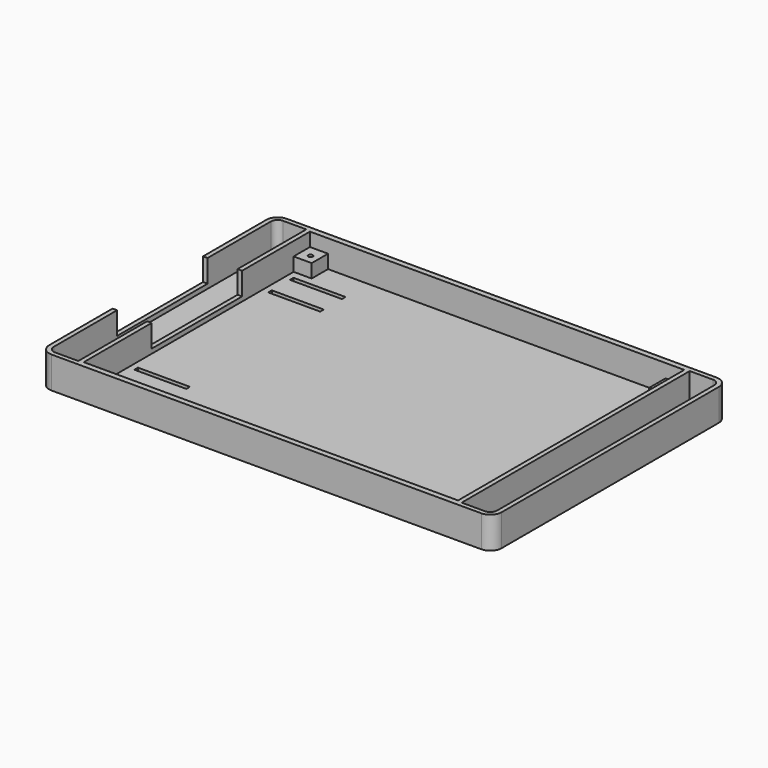
from build123d import *

# Parameters (mm, degrees)
F0_W         = 200
F0_H         = 130
F0_W_2       = 0.3
F0_H_2       = 106.96
F1_DEPTH     = 2
F2_DEPTH     = 14
F3_DEPTH     = 8
F4_D         = 2
F5_R         = 5
F6_T         = 2
F6_T3_DEPTH  = 16
F6_T5_DEPTH  = 10
F6_T7_DEPTH  = 12
F6_T9_DEPTH  = 10
F6_T11_DEPTH = 153.2
F6_T13_DEPTH = 12
F6_T15_DEPTH = 4.3
F6_T17_DEPTH = 129
F6_T19_DEPTH = 12.3
F6_T21_DEPTH = 11.7
F6_T23_DEPTH = 153.2
F6_T25_DEPTH = 13.02
F6_T27_DEPTH = 13.02
F6_T29_DEPTH = 110.96
F7_W         = 23
F7_H         = 2
F8_DEPTH     = 22.5
F9_W         = 50
F9_H         = 8
F9_H_2       = 2
F10_DEPTH    = 25


# Not quite as in the source:
# - a shell that OpenCascade refuses in one call is made with other operations: the cavity is built on its own and cut out


with BuildPart() as f1:
    # F0 (on Top) → F1 (new body)
    with BuildSketch(Plane.XY):
        Rectangle(F0_W, F0_H)
        Polygon((77.15, 62.5), (79.15, 62.5), (82.45, 62.5), (82.75, 62.5), (82.75, 59.5), (82.75, -58.77), (82.75, -62.5), (82.45, -62.5), (79.45, -62.5), (77.45, -62.5), (74.75, -62.5), (-74.45, -62.5), (-77.45, -62.5), (-79.45, -62.5), (-82.75, -62.5), (-82.75, -58.77), (-82.75, -53.48), (-82.75, 53.48), (-82.75, 59.5), (-82.75, 62.5), (-79.75, 62.5), (-77.75, 62.5), (-74.75, 62.5), (74.45, 62.5), align=None, mode=Mode.SUBTRACT)
        Polygon((74.45, 53.48), (74.45, 62.5), (-74.75, 62.5), (-74.75, 53.48), (-82.45, 53.48), (-82.45, -53.48), (-74.45, -53.48), (-74.45, -62.5), (74.75, -62.5), (74.75, -53.48), (82.45, -53.48), (82.45, 53.48), align=None)
        Polygon((-74.75, 53.48), (-74.75, 62.5), (-77.75, 62.5), (-79.75, 62.5), (-82.75, 62.5), (-82.75, 59.5), (-82.75, 53.48), (-82.45, 53.48), align=None)
        Polygon((82.45, 62.5), (79.15, 62.5), (77.15, 62.5), (74.45, 62.5), (74.45, 53.48), (82.45, 53.48), align=None)
        Polygon((82.45, -62.5), (82.45, -53.48), (74.75, -53.48), (74.75, -62.5), (77.45, -62.5), (79.45, -62.5), align=None)
        Polygon((-74.45, -53.48), (-82.45, -53.48), (-82.75, -53.48), (-82.75, -58.77), (-82.75, -62.5), (-79.45, -62.5), (-77.45, -62.5), (-74.45, -62.5), align=None)
        with Locations((-82.6, 0)):
            Rectangle(F0_W_2, F0_H_2)
        Polygon((82.75, 62.5), (82.45, 62.5), (82.45, 53.48), (82.45, -53.48), (82.45, -62.5), (82.75, -62.5), (82.75, -58.77), (82.75, 59.5), align=None)
    extrude(amount=F1_DEPTH)

    # F0 (on Top) → F2 (join)
    with BuildSketch(Plane.XY):
        Rectangle(F0_W, F0_H)
        Polygon((77.15, 62.5), (79.15, 62.5), (82.45, 62.5), (82.75, 62.5), (82.75, 59.5), (82.75, -58.77), (82.75, -62.5), (82.45, -62.5), (79.45, -62.5), (77.45, -62.5), (74.75, -62.5), (-74.45, -62.5), (-77.45, -62.5), (-79.45, -62.5), (-82.75, -62.5), (-82.75, -58.77), (-82.75, -53.48), (-82.75, 53.48), (-82.75, 59.5), (-82.75, 62.5), (-79.75, 62.5), (-77.75, 62.5), (-74.75, 62.5), (74.45, 62.5), align=None, mode=Mode.SUBTRACT)
    extrude(amount=F2_DEPTH)

    # F0 (on Top) → F3 (join)
    with BuildSketch(Plane.XY):
        Polygon((-74.45, -53.48), (-82.45, -53.48), (-82.75, -53.48), (-82.75, -58.77), (-82.75, -62.5), (-79.45, -62.5), (-77.45, -62.5), (-74.45, -62.5), align=None)
        Polygon((-74.75, 53.48), (-74.75, 62.5), (-77.75, 62.5), (-79.75, 62.5), (-82.75, 62.5), (-82.75, 59.5), (-82.75, 53.48), (-82.45, 53.48), align=None)
        Polygon((82.45, -62.5), (82.45, -53.48), (74.75, -53.48), (74.75, -62.5), (77.45, -62.5), (79.45, -62.5), align=None)
        Polygon((82.45, 62.5), (79.15, 62.5), (77.15, 62.5), (74.45, 62.5), (74.45, 53.48), (82.45, 53.48), align=None)
    extrude(amount=F3_DEPTH)

    # F4 (through all)
    with Locations(Plane(origin=(0, 0, 0), x_dir=(1, 0, 0), z_dir=(0, 0, -1))):
        with Locations((-78.45, 57.48), (78.45, 57.48), (-78.45, -57.48), (78.45, -57.48)):
            Hole(F4_D / 2)

    # F5
    f5_edges = [f1.edges().sort_by_distance(p)[0] for p in [
        (-100, -65, 7),
        (-100, 65, 7),
        (100, 65, 7),
        (100, -65, 7),
    ]]
    fillet(f5_edges, radius=F5_R)

    # F6: shell of thickness 2, made by hand


with BuildPart() as f6_core1:
    # F6_t2: copy of F1
    add(f1.part)

    # the walls: a layer under each face that stays
    f6_faces = [f6_core1.faces().sort_by_distance(p)[0] for p in [
        (100, 0, 7),
        (98.5355339059, -63.5355339059, 7),
        (98.5355339059, 63.5355339059, 7),
        (0, 0, 0),
        (0, -65, 7),
        (0, 65, 7),
        (-98.5355339059, -63.5355339059, 7),
        (-98.5355339059, 63.5355339059, 7),
        (-100, 0, 7),
        (0, 62.5, 8),
        (82.75, 0, 8),
        (0, -62.5, 8),
        (-82.75, 0, 8),
        (-79.45, -57.48, 4),
        (77.45, -57.48, 4),
        (-79.45, 57.48, 4),
        (77.45, 57.48, 4),
        (-81.4166666667, 54.9833333333, 8),
        (-74.75, 57.99, 5),
        (0, 0, 2),
        (74.45, 57.99, 5),
        (75.7833333333, 54.9833333333, 8),
        (82.45, 57.99, 5),
        (-74.45, -57.99, 5),
        (-81.3666666667, -60.9966666667, 8),
        (82.45, -57.99, 5),
        (76.0333333333, -60.9966666667, 8),
        (74.75, -57.99, 5),
        (-78.75, 53.48, 5),
        (-78.6, -53.48, 5),
        (78.6, -53.48, 5),
        (78.45, 53.48, 5),
    ]]
    thicken(f6_faces, amount=-F6_T, mode=Mode.SUBTRACT)

    # F6_s4 → F6_t3 (cut)
    with BuildSketch(Plane.XY):
        Polygon((82.73, 62.48), (82.75, 64.5), (84.75, 64.5), (84.75, 62.5), align=None)
        Polygon((82.73, -62.48), (84.75, -62.5), (84.75, -64.5), (82.75, -64.5), align=None)
    extrude(amount=F6_T3_DEPTH, mode=Mode.SUBTRACT)

    # F6_s6 → F6_t5 (cut)
    with BuildSketch(Plane.XY.offset(6)):
        Polygon((-82.73, 62.48), (-82.75, 64.5), (-84.75, 64.5), (-84.75, 62.5), align=None)
        Polygon((-82.73, -62.48), (-82.75, -64.5), (-84.75, -64.5), (-84.75, -62.5), align=None)
    extrude(amount=F6_T5_DEPTH, mode=Mode.SUBTRACT)

    # F6_s8 → F6_t7 (cut)
    with BuildSketch(Plane.YZ.offset(-84.75)):
        Polygon((62.48, 8.02), (64.5, 8), (64.5, 6), (62.5, 6), align=None)
        Polygon((53.46, 2.02), (53.48, 0), (55.48, 0), (55.48, 2), align=None)
    extrude(amount=F6_T7_DEPTH, mode=Mode.SUBTRACT)

    # F6_s10 → F6_t9 (cut)
    with BuildSketch(Plane.XY):
        Polygon((-74.73, 62.48), (-74.75, 64.5), (-76.75, 64.5), (-76.75, 62.5), align=None)
        Polygon((74.43, 62.48), (74.45, 64.5), (76.45, 64.5), (76.45, 62.5), align=None)
        Polygon((82.47, 62.48), (82.45, 64.5), (80.45, 64.5), (80.45, 62.5), align=None)
        Polygon((-74.43, -62.48), (-74.45, -64.5), (-76.45, -64.5), (-76.45, -62.5), align=None)
        Polygon((82.47, -62.48), (82.45, -64.5), (80.45, -64.5), (80.45, -62.5), align=None)
        Polygon((74.73, -62.48), (74.75, -64.5), (76.75, -64.5), (76.75, -62.5), align=None)
        Polygon((-82.73, 53.46), (-84.75, 53.48), (-84.75, 55.48), (-82.75, 55.48), align=None)
        Polygon((-82.73, -53.46), (-84.75, -53.48), (-84.75, -55.48), (-82.75, -55.48), align=None)
    extrude(amount=F6_T9_DEPTH, mode=Mode.SUBTRACT)

    # F6_s12 → F6_t11 (cut)
    with BuildSketch(Plane.YZ.offset(-76.75)):
        Polygon((62.48, 2.02), (64.5, 2), (64.5, 0), (62.5, 0), align=None)
    extrude(amount=F6_T11_DEPTH, mode=Mode.SUBTRACT)

    # F6_s14 → F6_t13 (cut)
    with BuildSketch(Plane.YZ.offset(72.45)):
        Polygon((62.48, 8.02), (64.5, 8), (64.5, 6), (62.5, 6), align=None)
        Polygon((53.46, 2.02), (53.48, 0), (55.48, 0), (55.48, 2), align=None)
    extrude(amount=F6_T13_DEPTH, mode=Mode.SUBTRACT)

    # F6_s16 → F6_t15 (cut)
    with BuildSketch(Plane.YZ.offset(80.45)):
        Polygon((62.48, 2.02), (64.5, 2), (64.5, 0), (62.5, 0), align=None)
        Polygon((-62.48, 2.02), (-64.5, 2), (-64.5, 0), (-62.5, 0), align=None)
    extrude(amount=F6_T15_DEPTH, mode=Mode.SUBTRACT)

    # F6_s18 → F6_t17 (cut)
    with BuildSketch(Plane.XZ.offset(-64.5)):
        Polygon((82.73, 2.02), (84.75, 2), (84.75, 0), (82.75, 0), align=None)
    extrude(amount=F6_T17_DEPTH, mode=Mode.SUBTRACT)

    # F6_s20 → F6_t19 (cut)
    with BuildSketch(Plane.YZ.offset(-84.75)):
        Polygon((-62.48, 8.02), (-64.5, 8), (-64.5, 6), (-62.5, 6), align=None)
        Polygon((-53.46, 2.02), (-53.48, 0), (-55.48, 0), (-55.48, 2), align=None)
    extrude(amount=F6_T19_DEPTH, mode=Mode.SUBTRACT)

    # F6_s22 → F6_t21 (cut)
    with BuildSketch(Plane.YZ.offset(72.75)):
        Polygon((-62.48, 8.02), (-64.5, 8), (-64.5, 6), (-62.5, 6), align=None)
        Polygon((-53.46, 2.02), (-53.48, 0), (-55.48, 0), (-55.48, 2), align=None)
    extrude(amount=F6_T21_DEPTH, mode=Mode.SUBTRACT)

    # F6_s24 → F6_t23 (cut)
    with BuildSketch(Plane.YZ.offset(-76.45)):
        Polygon((-62.48, 2.02), (-64.5, 2), (-64.5, 0), (-62.5, 0), align=None)
    extrude(amount=F6_T23_DEPTH, mode=Mode.SUBTRACT)

    # F6_s26 → F6_t25 (cut)
    with BuildSketch(Plane.XZ.offset(-64.5)):
        Polygon((-82.73, 8.02), (-84.75, 8), (-84.75, 6), (-82.75, 6), align=None)
        Polygon((-74.73, 2.02), (-76.75, 2), (-76.75, 0), (-74.75, 0), align=None)
        Polygon((74.43, 2.02), (74.45, 0), (76.45, 0), (76.45, 2), align=None)
        Polygon((82.47, 2.02), (82.45, 0), (80.45, 0), (80.45, 2), align=None)
    extrude(amount=F6_T25_DEPTH, mode=Mode.SUBTRACT)

    # F6_s28 → F6_t27 (cut)
    with BuildSketch(Plane.XZ.offset(51.48)):
        Polygon((-82.73, 8.02), (-84.75, 8), (-84.75, 6), (-82.75, 6), align=None)
        Polygon((82.47, 2.02), (82.45, 0), (80.45, 0), (80.45, 2), align=None)
        Polygon((74.73, 2.02), (74.75, 0), (76.75, 0), (76.75, 2), align=None)
        Polygon((-74.43, 2.02), (-74.45, 0), (-76.45, 0), (-76.45, 2), align=None)
    extrude(amount=F6_T27_DEPTH, mode=Mode.SUBTRACT)

    # F6_s30 → F6_t29 (cut)
    with BuildSketch(Plane.XZ.offset(-55.48)):
        Polygon((-82.73, 2.02), (-84.75, 2), (-84.75, 0), (-82.75, 0), align=None)
    extrude(amount=F6_T29_DEPTH, mode=Mode.SUBTRACT)


with BuildPart() as f1_1:
    add(f1.part)

    # what is left inside the walls is the cavity
    f6_cavity = [f6_core1.part.solids().sort_by_distance(p)[0] for p in [
        (91.375, -21, 13.98),
        (-87.225, -21, 2.02),
        (78.642053, -60.493887, 4.666667),
        (78.45, 60.5, 4.666667),
    ]]
    add(f6_cavity, mode=Mode.SUBTRACT)

    # F7 (on face) → F8 (cut)
    with BuildSketch(Plane(origin=(0, 0, 0), x_dir=(1, 0, 0), z_dir=(0, 0, -1))):
        with Locations((-68.5, 49)):
            Rectangle(F7_W, F7_H)
        with Locations((-68.5, 37)):
            Rectangle(F7_W, F7_H)
        with Locations((-68.5, -37)):
            Rectangle(F7_W, F7_H)
        with Locations((-68.5, -49)):
            Rectangle(F7_W, F7_H)
    extrude(amount=-F8_DEPTH, mode=Mode.SUBTRACT)

    # F9 (on face) → F10 (cut)
    with BuildSketch(Plane.YZ.offset(-82.75)):
        with Locations((0, 8)):
            Rectangle(F9_W, F9_H)
        with Locations((0, 13)):
            Rectangle(F9_W, F9_H_2)
    extrude(amount=-F10_DEPTH, mode=Mode.SUBTRACT)


solid = f1_1.part
